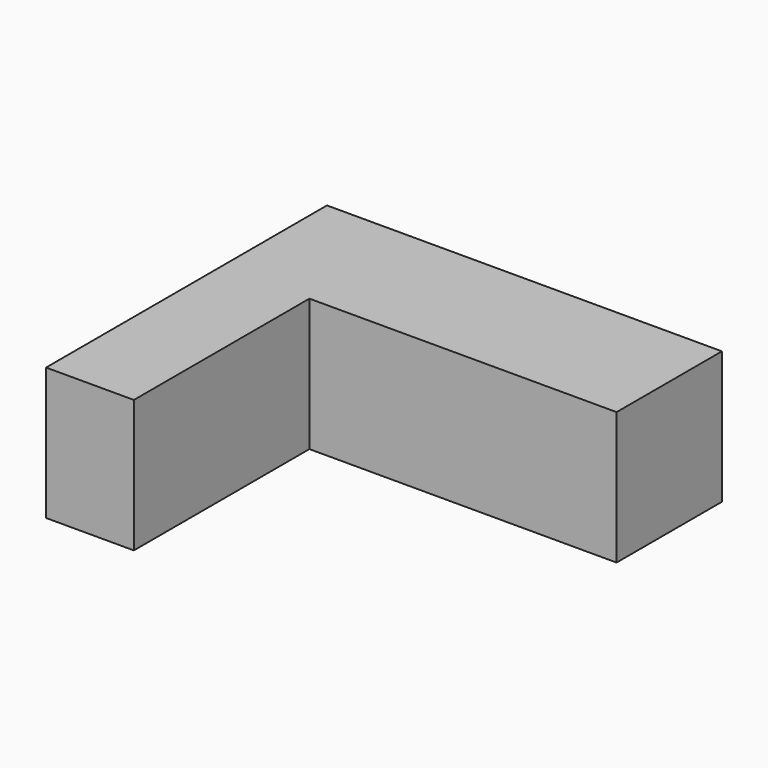
from build123d import *

# Parameters (mm, degrees)
F1_DEPTH = 500


with BuildPart() as f1:
    # F0 (on Top) → F1 (new body)
    with BuildSketch(Plane.XY):
        Polygon((-1005.9320986634, 1669.9280071504), (-2496.6424078943, 1669.9280071504), (-2496.6424078943, 344.852176723), (-2165.3734502874, 344.852176723), (-2165.3734502874, 1173.0245707402), (-1005.9320986634, 1173.0245707402), align=None)
    extrude(amount=F1_DEPTH)


solid = f1.part
